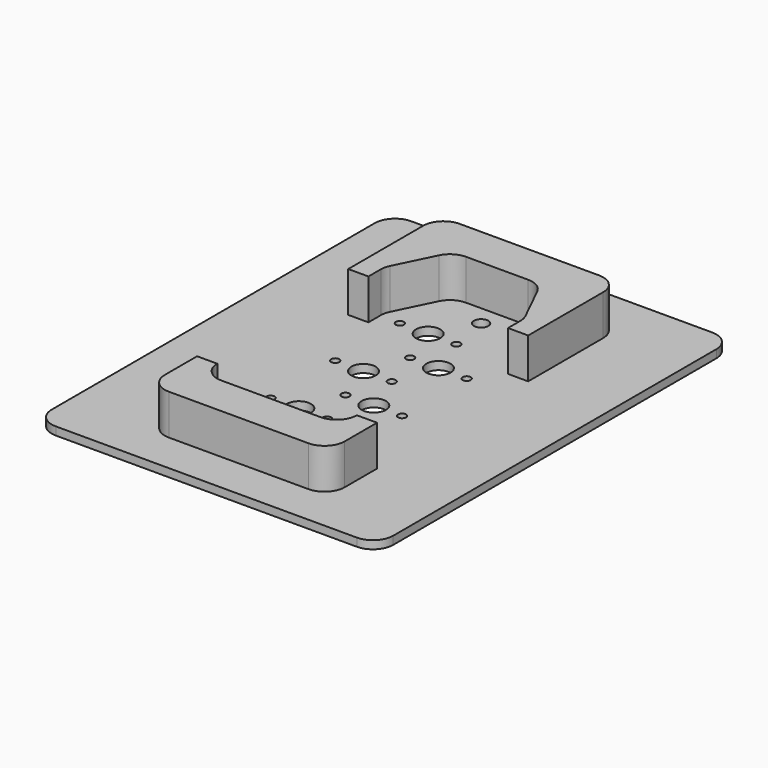
from build123d import *

# Parameters (mm, degrees)
F0_W     = 84.554
F0_H     = 110
F0_R     = 3
F0_R_2   = 1.778
F1_DEPTH = 2
F2_DEPTH = 12
F3_DEPTH = 12
F4_R     = 4.99999
F5_R     = 5
F6_R     = 1
F7_DEPTH = 25
F8_DEPTH = 25


# Not quite as in the source:
# - a fillet or chamfer is up to 0.001 mm smaller than in the source, because OpenCascade refuses the exact size
# - a feature names something its author has since deleted; it is built from what else it names


with BuildPart() as f1:
    # F0 (on Top) → F1 (new body)
    with BuildSketch(Plane.XY):
        with Locations((17.277, 35)):
            Rectangle(F0_W, F0_H)
        with Locations((12, 15.25)):
            Circle(F0_R, mode=Mode.SUBTRACT)
        Polygon((0, 5), (0, 0), (34.554, 0), (34.554, 5), (39.554, 5), (39.554, -10), (-5, -10), (-5, 5), align=None, mode=Mode.SUBTRACT)
        with Locations((17.277, 4.95)):
            Circle(F0_R_2, mode=Mode.SUBTRACT)
        with Locations((22.554, 25.25)):
            Circle(F0_R, mode=Mode.SUBTRACT)
        with Locations((12, 35.25)):
            Circle(F0_R, mode=Mode.SUBTRACT)
        with Locations((12, 55.25)):
            Circle(F0_R, mode=Mode.SUBTRACT)
        with Locations((22.554, 45.25)):
            Circle(F0_R, mode=Mode.SUBTRACT)
        with Locations((17.277, 65.05)):
            Circle(F0_R_2, mode=Mode.SUBTRACT)
        Polygon((6.482, 70), (0, 56.776), (0, 51.776), (-5, 51.776), (-5, 80), (39.554, 80), (39.554, 51.776), (34.554, 51.776), (34.554, 56.776), (28.072, 70), align=None, mode=Mode.SUBTRACT)
    extrude(amount=F1_DEPTH)

    # F0 (on Top) → F2 (join)
    with BuildSketch(Plane.XY):
        Polygon((0, 51.776), (0, 56.776), (6.482, 70), (28.072, 70), (34.554, 56.776), (34.554, 51.776), (39.554, 51.776), (39.554, 80), (-5, 80), (-5, 51.776), align=None)
    extrude(amount=F2_DEPTH)

    # F0 (on Top) → F3 (join)
    with BuildSketch(Plane.XY):
        Polygon((34.554, 0), (0, 0), (0, 5), (-5, 5), (-5, -10), (39.554, -10), (39.554, 5), (34.554, 5), align=None)
    extrude(amount=F3_DEPTH)

    # F4 (radius 5 in the source; OpenCascade refuses exactly that, so slightly less here)
    f4_edges = [f1.edges().sort_by_distance(p)[0] for p in [
        (6.482, 70, 7),
        (28.072, 70, 7),
        (0, 56.776, 7),
        (34.554, 56.776, 7),
        (34.554, 0, 7),
        (0, 0, 7),
        (59.554, -20, 1),
        (59.554, 90, 1),
        (-25, 90, 1),
        (-25, -20, 1),
    ]]
    fillet(f4_edges, radius=F4_R)

    # F5
    f5_edges = [f1.edges().sort_by_distance(p)[0] for p in [
        (-5, -10, 7),
        (39.554, -10, 7),
        (39.554, 80, 7),
        (-5, 80, 7),
    ]]
    fillet(f5_edges, radius=F5_R)

    # F6 (on face) → F7 (cut)
    with BuildSketch(Plane.XY.offset(2)):
        with Locations((5, 55.25)):
            Circle(F6_R)
        with Locations((19, 55.25)):
            Circle(F6_R)
        with Locations((19, 35.25)):
            Circle(F6_R)
        with Locations((5, 35.25)):
            Circle(F6_R)
        with Locations((15.554, 25.25)):
            Circle(F6_R)
        with Locations((29.554, 25.25)):
            Circle(F6_R)
    extrude(amount=-F7_DEPTH, mode=Mode.SUBTRACT)

    # F6 (on face) → F8 (cut)
    with BuildSketch(Plane.XY.offset(2)):
        with Locations((5, 55.25)):
            Circle(F6_R)
        with Locations((19, 55.25)):
            Circle(F6_R)
        with Locations((19, 35.25)):
            Circle(F6_R)
        with Locations((5, 35.25)):
            Circle(F6_R)
        with Locations((15.554, 25.25)):
            Circle(F6_R)
        with Locations((29.554, 25.25)):
            Circle(F6_R)
        with Locations((15.554, 45.25)):
            Circle(F6_R)
        with Locations((29.554, 45.25)):
            Circle(F6_R)
        with Locations((5, 15.25)):
            Circle(F6_R)
        with Locations((19, 15.25)):
            Circle(F6_R)
    extrude(amount=-F8_DEPTH, mode=Mode.SUBTRACT)


solid = f1.part
